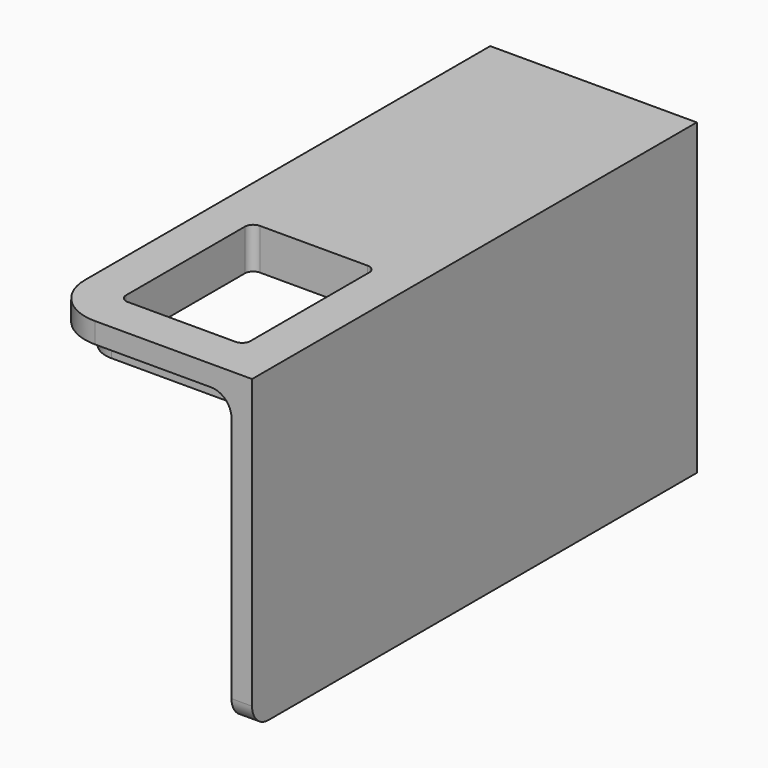
from build123d import *

# Parameters (mm, degrees)
F1_DEPTH = 5
F2_DEPTH = 10
F3_DEPTH = 75
F4_R     = 4.99999


# Not quite as in the source:
# - a fillet or chamfer is up to 0.001 mm smaller than in the source, because OpenCascade refuses the exact size


with BuildPart() as f1:
    # F0 (on Top) → F1 (new body)
    with BuildSketch(Plane.XY):
        with BuildLine():
            ThreePointArc((-20.1, 18.05), (-18.0497474683, 22.9997474683), (-13.1, 25.05))
            Line((-13.1, 25.05), (20.1, 25.05))
            Line((20.1, 25.05), (20.1, 100.05))
            Line((20.1, 100.05), (-25.1, 100.05))
            Line((-25.1, 100.05), (-25.1, -18.05))
            ThreePointArc((-25.1, -18.05), (-21.5852813742, -26.5352813742), (-13.1, -30.05))
            Line((-13.1, -30.05), (20.1, -30.05))
            Line((20.1, -30.05), (20.1, -25.05))
            Line((20.1, -25.05), (-13.1, -25.05))
            ThreePointArc((-13.1, -25.05), (-18.0497474683, -22.9997474683), (-20.1, -18.05))
            Line((-20.1, -18.05), (-20.1, 18.05))
        make_face()
    extrude(amount=-F1_DEPTH)

    # F0 (on Top) → F2 (join)
    with BuildSketch(Plane.XY):
        with BuildLine():
            Line((20.1, 25.05), (-13.1, 25.05))
            ThreePointArc((-13.1, 25.05), (-18.0497474683, 22.9997474683), (-20.1, 18.05))
            Line((-20.1, 18.05), (-20.1, -18.05))
            ThreePointArc((-20.1, -18.05), (-18.0497474683, -22.9997474683), (-13.1, -25.05))
            Line((-13.1, -25.05), (20.1, -25.05))
            Line((20.1, -25.05), (20.1, 25.05))
        make_face()
        with BuildLine():
            Line((-13.1, 20.05), (13.1, 20.05))
            ThreePointArc((13.1, 20.05), (14.5142135624, 19.4642135624), (15.1, 18.05))
            Line((15.1, 18.05), (15.1, -18.05))
            ThreePointArc((15.1, -18.05), (14.5142135624, -19.4642135624), (13.1, -20.05))
            Line((13.1, -20.05), (-13.1, -20.05))
            ThreePointArc((-13.1, -20.05), (-14.5142135624, -19.4642135624), (-15.1, -18.05))
            Line((-15.1, -18.05), (-15.1, 18.05))
            ThreePointArc((-15.1, 18.05), (-14.5142135624, 19.4642135624), (-13.1, 20.05))
        make_face(mode=Mode.SUBTRACT)
    extrude(amount=-F2_DEPTH)

    # F0 (on Top) → F3 (join)
    with BuildSketch(Plane.XY):
        Polygon((20.1, 100.05), (20.1, 25.05), (20.1, -25.05), (20.1, -30.05), (25.1, -30.05), (25.1, 105.05), (-25.1, 105.05), (-25.1, 100.05), align=None)
    extrude(amount=-F3_DEPTH)

    # F4 (radius 5 in the source; OpenCascade refuses exactly that, so slightly less here)
    f4_edges = [f1.edges().sort_by_distance(p)[0] for p in [
        (20.1, -27.55, -5),
        (20.1, 62.55, -5),
        (20.1, 0, -10),
        (22.6, -30.05, -75),
        (-25.1, 102.55, -75),
        (-2.5, 100.05, -5),
    ]]
    fillet(f4_edges, radius=F4_R)


solid = f1.part
